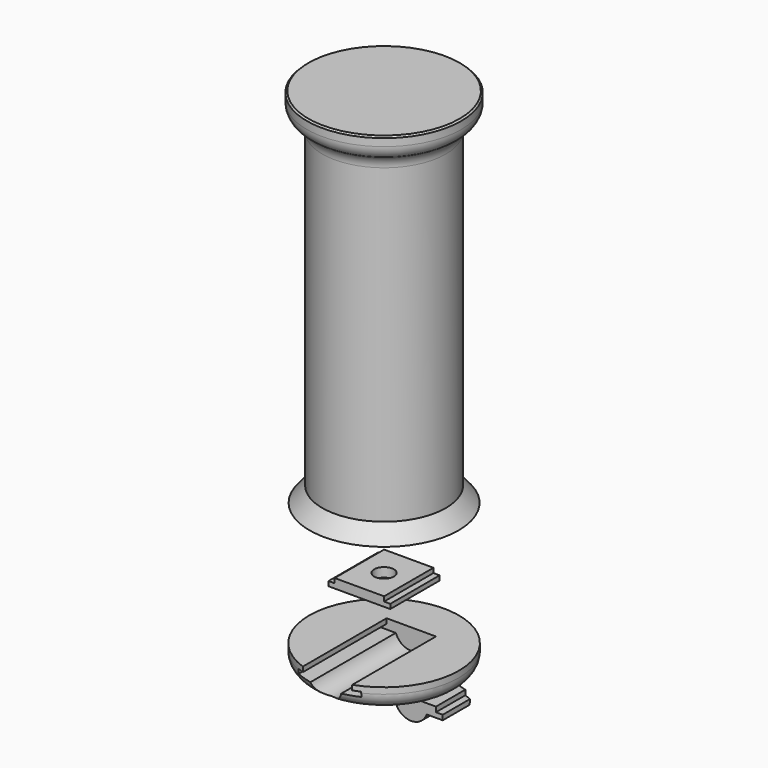
from build123d import *

# Parameters (mm, degrees)
F2_SIZE     = 2
F4_SIZE     = 1
F5_SIZE     = 0.5
F6_R        = 25
F6_R_2      = 20
F7_DEPTH    = 5
F8_S5_R     = 20
F8_T6_DEPTH = 37
F10_W       = 20
F10_H       = 20
F10_R       = 3.2
F11_DEPTH   = 3
F12_W       = 2
F12_H       = 1.5
F13_DEPTH   = 10
F15_R       = 24.25
F16_DEPTH   = 7
F17_R       = 5
F19_DEPTH   = 25
F20_DEPTH   = 11
F23_DEPTH   = 50


# Not quite as in the source:
# - a fillet or chamfer that OpenCascade refuses, or shapes differently, is made with other operations: its cross-section is extruded or revolved along the edge and cut away or added


with BuildPart() as f1:
    # F0 (on Front) → F1 (revolve)
    with BuildSketch(Plane.XZ):
        Polygon((3, 40), (3, 0), (20, 0), (20, 110), (25, 110), (25, 117.5), (0, 117.5), (0, 40), align=None)
    revolve(axis=Axis((0, 0, 78.75), (0, 0, -1)))

    # F2
    f2_edges = [f1.edges().sort_by_distance(p)[0] for p in [
        (-20, 0, 110),
    ]]
    chamfer(f2_edges, length=F2_SIZE)

    # F3: fillet of radius 5 on 2 edges, made by hand

    # F3_s1 → F3_t2 (revolve)
    with BuildSketch(Plane.XZ):
        with BuildLine():
            ThreePointArc((20, 105.9289321881), (20.3806023374, 107.84234935), (21.4644660941, 109.4644660941))
            Line((21.4644660941, 109.4644660941), (20, 108))
            Line((20, 108), (20, 105.9289321881))
        make_face()
    revolve(axis=Axis((0, 0, 108), (0, 0, -1)))

    # F3_s3 → F3_t4 (revolve, cut)
    with BuildSketch(Plane.XZ):
        with BuildLine():
            ThreePointArc((22, 110), (24.1833001327, 111.8439629074), (25, 114.582575695))
            Line((25, 114.582575695), (25, 110))
            Line((25, 110), (22, 110))
        make_face()
    revolve(axis=Axis((0, 0, 110), (0, 0, -1)), mode=Mode.SUBTRACT)

    # F4
    f4_edges = [f1.edges().sort_by_distance(p)[0] for p in [
        (-3, 0, 0),
    ]]
    chamfer(f4_edges, length=F4_SIZE)

    # F5
    f5_edges = [f1.edges().sort_by_distance(p)[0] for p in [
        (-25, 0, 117.5),
    ]]
    chamfer(f5_edges, length=F5_SIZE)

    # F6 (on Top) → F7 (join)
    with BuildSketch(Plane.XY):
        Circle(F6_R)
        Circle(F6_R_2, mode=Mode.SUBTRACT)
    extrude(amount=F7_DEPTH)

    # F8: chamfer of 5 x 6 on 1 edges, made by hand


with BuildPart() as f8_tool2:
    # F8_s3 → F8_t4 (revolve)
    with BuildSketch(Plane.XZ):
        Polygon((20, 5), (25, -1), (25, 5), align=None)
    revolve(axis=Axis((0, 0, 5), (0, 0, 1)))

    # F8_s5 → F8_t6 (cut, symmetric)
    with BuildSketch(Plane.XY.offset(2)):
        Circle(F8_S5_R)
    extrude(amount=F8_T6_DEPTH, both=True, mode=Mode.SUBTRACT)


with BuildPart() as f1_1:
    add(f1.part)

    # F8_t1: cut F8_tool2
    add(f8_tool2.part, mode=Mode.SUBTRACT)


with BuildPart() as f11:
    # F10 (on offset) → F11 (new body)
    with BuildSketch(Plane.XY.offset(-20)):
        Rectangle(F10_W, F10_H)
        Circle(F10_R, mode=Mode.SUBTRACT)
    extrude(amount=-F11_DEPTH)

    # F12 (on Front) → F13 (cut, symmetric)
    with BuildSketch(Plane.XZ):
        with Locations((-9, -20.75)):
            Rectangle(F12_W, F12_H)
        with Locations((9, -20.75)):
            Rectangle(F12_W, F12_H)
    extrude(amount=F13_DEPTH, both=True, mode=Mode.SUBTRACT)


with BuildPart() as f16:
    # F15 (on offset) → F16 (new body)
    with BuildSketch(Plane.XY.offset(-40)):
        Circle(F15_R)
    extrude(amount=-F16_DEPTH)

    # F17
    f17_edges = [f16.edges().sort_by_distance(p)[0] for p in [
        (-24.25, 0, -47),
    ]]
    fillet(f17_edges, radius=F17_R)

    # F18 (on Front) → F19 (cut)
    with BuildSketch(Plane.XZ):
        Polygon((0, -43.2), (0, -40), (-8, -40), (-8, -41.6), (-10.2, -41.6), (-10.2, -43.2), (-5, -43.2), align=None)
        Polygon((8, -40), (0, -40), (0, -43.2), (5, -43.2), (10.2, -43.2), (10.2, -41.6), (8, -41.6), align=None)
        with BuildLine():
            Line((5, -43.2), (0, -43.2))
            Line((0, -43.2), (-5, -43.2))
            ThreePointArc((-5, -43.2), (0, -46.7), (5, -43.2))
        make_face()
    extrude(amount=F19_DEPTH, mode=Mode.SUBTRACT)

    # F20 (cut): a face of the model
    f20_faces = [f16.faces().sort_by_distance(p)[0] for p in [
        (0, 0, -42.595240959),
    ]]
    extrude(f20_faces, amount=-F20_DEPTH, mode=Mode.SUBTRACT)


with BuildPart() as f21_1:
    # F21: copy of F16
    add(f16.part.moved(Location((0, 0, -20))))

    # F22 (on face) → F23 (cut, symmetric)
    with BuildSketch(Plane.XZ.offset(-11)):
        with BuildLine():
            Line((31.9885127246, -60), (8, -60))
            Line((8, -60), (8, -61.6))
            Line((8, -61.6), (10.2, -61.6))
            Line((10.2, -61.6), (10.2, -63.2))
            Line((10.2, -63.2), (5, -63.2))
            ThreePointArc((5, -63.2), (0, -66.7), (-5, -63.2))
            Line((-5, -63.2), (-10.2, -63.2))
            Line((-10.2, -63.2), (-10.2, -61.6))
            Line((-10.2, -61.6), (-8, -61.6))
            Line((-8, -61.6), (-8, -60))
            Line((-8, -60), (-32.2001688182, -60))
            Line((-32.2001688182, -60), (-32.2001688182, -71.0251182318))
            Line((-32.2001688182, -71.0251182318), (31.9885127246, -71.0251182318))
            Line((31.9885127246, -71.0251182318), (31.9885127246, -60))
        make_face()
    extrude(amount=F23_DEPTH, both=True, mode=Mode.SUBTRACT)


solid = Compound([f1_1.part, f11.part, f16.part, f21_1.part])
